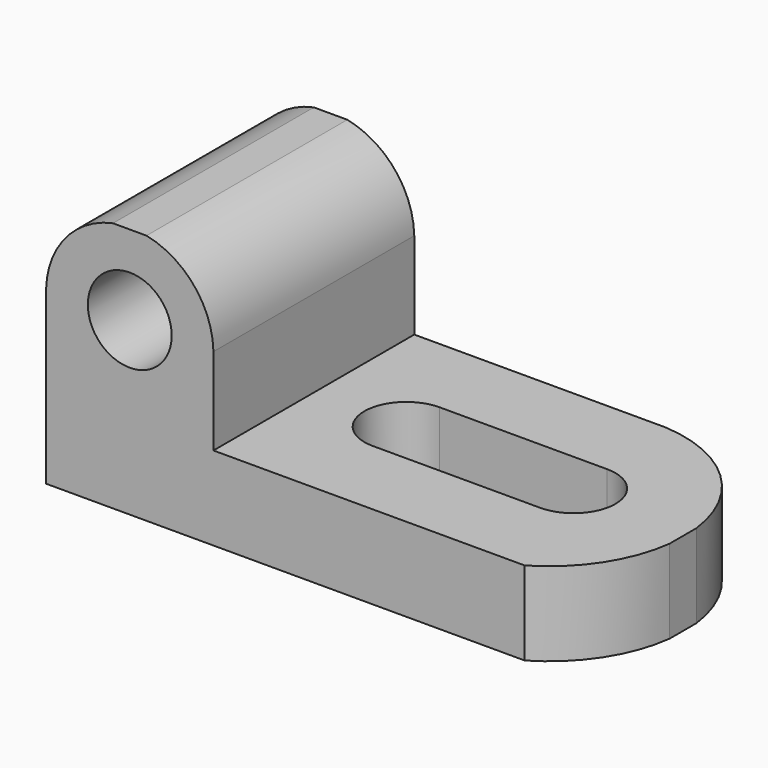
from build123d import *

# Parameters (mm, degrees)
F0_W      = 82.55
F0_H      = 38.1
F1_DEPTH  = 38.1
F2_W      = 57.15
F2_H      = 25.4
F3_DEPTH  = 38.101
F4_R      = 6.3636745149
F5_DEPTH  = 38.101
F7_DEPTH  = 25.4
F9_DEPTH  = 25.4
F10_DEPTH = 63.501
F12_DEPTH = 25.4


with BuildPart() as f1:
    # F0 (on Front) → F1 (new body)
    with BuildSketch(Plane.XZ):
        with Locations((-41.275, 19.05)):
            Rectangle(F0_W, F0_H)
    extrude(amount=F1_DEPTH)

    # F2 (on face) → F3 (cut, through all)
    with BuildSketch(Plane.XZ.offset(38.1)):
        with Locations((-28.575, 25.4)):
            Rectangle(F2_W, F2_H)
    extrude(amount=-F3_DEPTH, mode=Mode.SUBTRACT)

    # F4 (on face) → F5 (cut, through all)
    with BuildSketch(Plane.XZ.offset(38.1)):
        with Locations((-69.85, 25.9895079914)):
            Circle(F4_R)
    extrude(amount=-F5_DEPTH, mode=Mode.SUBTRACT)

    # F6 (on face) → F7 (cut)
    with BuildSketch(Plane.XY.offset(12.7)):
        with BuildLine():
            ThreePointArc((-43.1306947993, -12.7), (-38.6405667387, -14.5598719395), (-36.7806947993, -19.05))
            ThreePointArc((-36.7806947993, -19.05), (-38.6405667387, -23.5401280605), (-43.1306947993, -25.4))
            Line((-43.1306947993, -25.4), (-17.7306947993, -25.4))
            ThreePointArc((-17.7306947993, -25.4), (-24.0806947993, -19.05), (-17.7306947993, -12.7))
            Line((-17.7306947993, -12.7), (-43.1306947993, -12.7))
        make_face()
        with BuildLine():
            ThreePointArc((-43.1306947993, -25.4), (-38.6405667387, -23.5401280605), (-36.7806947993, -19.05))
            ThreePointArc((-36.7806947993, -19.05), (-38.6405667387, -14.5598719395), (-43.1306947993, -12.7))
            ThreePointArc((-43.1306947993, -12.7), (-49.4806947993, -19.05), (-43.1306947993, -25.4))
        make_face()
        with BuildLine():
            ThreePointArc((-11.3806947993, -19.05), (-13.2405667387, -14.5598719395), (-17.7306947993, -12.7))
            ThreePointArc((-17.7306947993, -12.7), (-24.0806947993, -19.05), (-17.7306947993, -25.4))
            ThreePointArc((-17.7306947993, -25.4), (-13.2405667387, -23.5401280605), (-11.3806947993, -19.05))
        make_face()
    extrude(amount=-F7_DEPTH, mode=Mode.SUBTRACT)

    # F8 (on face) → F9 (join)
    with BuildSketch(Plane.XZ.offset(38.1)):
        with BuildLine():
            ThreePointArc((-67.3090244137, 38.1), (-60.0909334069, 33.7845859546), (-57.15, 25.9058457722))
            Line((-57.15, 25.9058457722), (-57.15, 38.1))
            Line((-57.15, 38.1), (-67.3090244137, 38.1))
        make_face()
        with BuildLine():
            ThreePointArc((-82.55, 26.0334052145), (-79.5712875843, 33.8335010618), (-72.3941565633, 38.1))
            Line((-72.3941565633, 38.1), (-82.55, 38.1))
            Line((-82.55, 38.1), (-82.55, 26.0334052145))
        make_face()
    extrude(amount=F9_DEPTH)

    # F10 (cut, through all): faces of the model
    f10_faces = [f1.faces().sort_by_distance(p)[0] for p in [
        (-59.7492259595, -63.5, 35.2812720031),
        (-79.9507979007, -63.5, 35.2852151474),
    ]]
    extrude(f10_faces, amount=-F10_DEPTH, mode=Mode.SUBTRACT)

    # F11 (on face) → F12 (cut)
    with BuildSketch(Plane.XY.offset(12.7)):
        with BuildLine():
            ThreePointArc((-18.9558640122, 0), (-6.26601343, -5.5476288842), (0, -17.8985628462))
            Line((0, -17.8985628462), (0, 0))
            Line((0, 0), (-18.9558640122, 0))
        make_face()
        with BuildLine():
            ThreePointArc((0, -23.0064517831), (-3.2034542821, -31.7030229504), (-9.9095078185, -38.1))
            Line((-9.9095078185, -38.1), (0, -38.1))
            Line((0, -38.1), (0, -23.0064517831))
        make_face()
    extrude(amount=-F12_DEPTH, mode=Mode.SUBTRACT)


solid = f1.part
